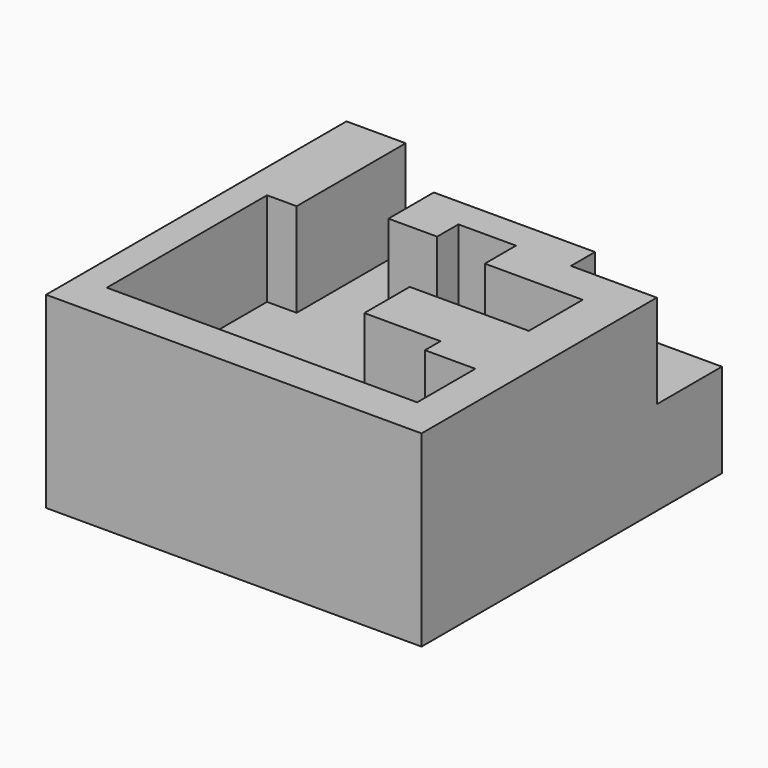
from build123d import *

# Parameters (mm, degrees)
F0_W     = 101.6
F0_H     = 101.6
F1_DEPTH = 25.4
F2_W     = 9.6067792356
F2_H     = 19.6575643495
F2_W_2   = 23.4931828454
F2_H_2   = 10.5259682656
F2_W_3   = 8.0198350638
F2_H_3   = 12.465775013
F2_H_4   = 41.7123902589
F2_W_4   = 11.6157357857
F2_H_5   = 18.2192062081
F3_DEPTH = 25.4


# Not quite as in the source:
# - ends of sketch curves that miss each other by under 0.0002 mm in the source are joined


with BuildPart() as f1:
    # F0 (on Top) → F1 (new body)
    with BuildSketch(Plane.XY):
        with Locations((2.876713872, 11.2423545628)):
            Rectangle(F0_W, F0_H)
    extrude(amount=F1_DEPTH)

    # F2 (on face) → F3 (join)
    with BuildSketch(Plane.XY.offset(25.4)):
        Polygon((-31.8836160004, 25.1464881003), (-31.8836160004, 62.0423545628), (-47.923286128, 62.0423545628), (-47.923286128, 25.1464881003), (-39.9034510642, 25.1464881003), align=None)
        Polygon((0, 32.8177288175), (0, 40.0095209479), (0, 48.1602139771), (-13.1849600002, 48.1602139771), (-13.1849600002, 32.8177288175), align=None)
        Polygon((15.5822057277, 40.0095209479), (30.4452423006, 40.0095209479), (30.4452423006, 48.1602139771), (0, 48.1602139771), (0, 40.0095209479), align=None)
        Polygon((42.0609780863, 29.4615607709), (53.676713872, 29.4615607709), (53.676713872, 40.0095209479), (30.4452423006, 40.0095209479), (15.5822057277, 40.0095209479), (15.5822057277, 29.4615607709), align=None)
        Polygon((30.4452423006, -4.1001341306), (30.4452423006, 11.2423545628), (9.8287723958, 11.2423505634), (9.8287723958, -4.1001341306), align=None)
        Polygon((44.0699346364, -9.3741128221), (53.676713872, -9.3741128221), (53.676713872, 11.2423545628), (42.0609780863, 11.2423545628), (30.4452423006, 11.2423545628), (30.4452423006, -4.1001341306), (30.4452423006, -9.3741128221), (42.0609780863, -9.3741128221), align=None)
        with Locations((48.8733242542, -19.2028949969)):
            Rectangle(F2_W, F2_H)
        Polygon((53.676713872, -39.5576454372), (53.676713872, -29.0316771716), (44.0699346364, -29.0316771716), (42.0609780863, -29.0316771716), (-8.390433155, -29.0316771716), (-8.390433155, -39.5576454372), align=None)
        with Locations((-20.1370245777, -34.2946613044)):
            Rectangle(F2_W_2, F2_H_2)
        with Locations((-43.9133685961, -22.7987896651)):
            Rectangle(F2_W_3, F2_H_3)
        Polygon((-47.923286128, -39.5576454372), (-31.8836160004, -39.5576454372), (-31.8836160004, -29.0316771716), (-39.9034510642, -29.0316771716), (-47.923286128, -29.0316771716), align=None)
        with Locations((-43.9133685961, 4.2902929708)):
            Rectangle(F2_W_3, F2_H_4)
        with Locations((47.8688459791, 20.3519576668)):
            Rectangle(F2_W_4, F2_H_5)
    extrude(amount=F3_DEPTH)


solid = f1.part
